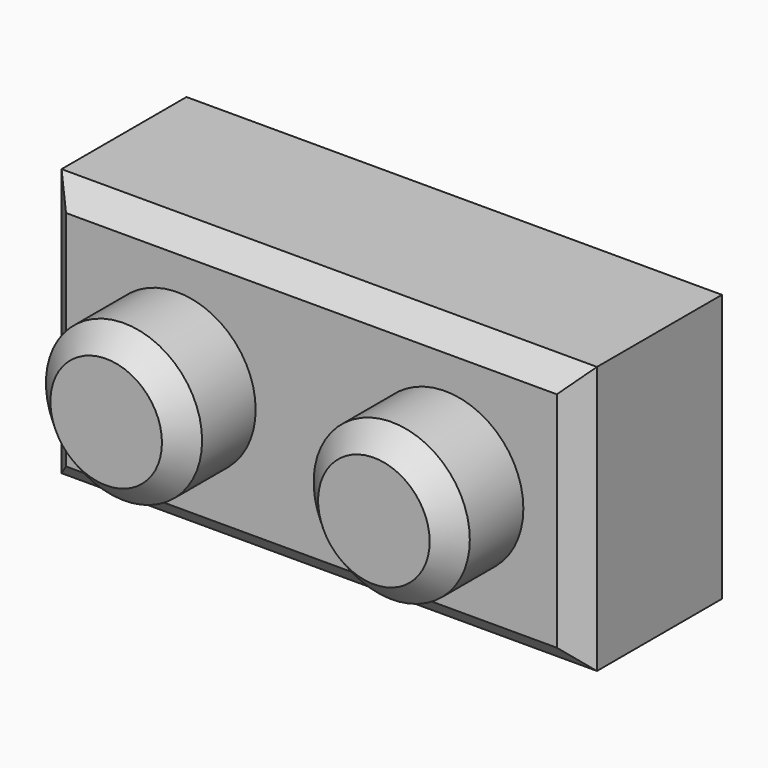
from build123d import *

# Parameters (mm, degrees)
F0_W     = 76.2
F0_H     = 38.1
F1_DEPTH = 25.4
F2_R     = 11.1125
F3_DEPTH = 12.7
F4_SIZE2 = 3.175
F4_SIZE  = 3.175
F5_SIZE2 = 3.175
F5_SIZE  = 3.175
F6_SIZE2 = 3.175
F6_SIZE  = 3.175
F7_T     = 7.9375


# Not quite as in the source:
# - a shell that OpenCascade refuses in one call is made with other operations: the cavity is built on its own and cut out


with BuildPart() as f1:
    # F0 (on Front) → F1 (new body)
    with BuildSketch(Plane.XZ):
        Rectangle(F0_W, F0_H)
    extrude(amount=F1_DEPTH)

    # F2 (on face) → F3 (join)
    with BuildSketch(Plane.XZ.offset(25.4)):
        with Locations((-19.05, 0)):
            Circle(F2_R)
        with Locations((19.05, 0)):
            Circle(F2_R)
    extrude(amount=F3_DEPTH)

    # F4
    f4_edges = [f1.edges().sort_by_distance(p)[0] for p in [
        (7.9375, -38.1, 0),
        (-30.1625, -38.1, 0),
    ]]
    chamfer(f4_edges, length=F4_SIZE, length2=F4_SIZE2)

    # F5
    f5_edges = [f1.edges().sort_by_distance(p)[0] for p in [
        (0, -25.4, 19.05),
    ]]
    chamfer(f5_edges, length=F5_SIZE, length2=F5_SIZE2)

    # F6
    f6_edges = [f1.edges().sort_by_distance(p)[0] for p in [
        (38.1, -25.4, -1.5875),
        (0, -25.4, -19.05),
        (-38.1, -25.4, -1.5875),
    ]]
    chamfer(f6_edges, length=F6_SIZE, length2=F6_SIZE2)

    # F7: shell of thickness 7.9375, made by hand


with BuildPart() as f7_core1:
    # F7_t2: copy of F1
    add(f1.part)

    # the walls: a layer under each face that stays
    f7_faces = [f7_core1.faces().sort_by_distance(p)[0] for p in [
        (0, -25.4, 0),
        (0, -23.8125, 17.4625),
        (36.5125, -23.8125, 0),
        (-36.5125, -23.8125, 0),
        (0, -23.8125, -17.4625),
        (-30.1625, -30.1625, 0),
        (7.9375, -30.1625, 0),
        (0, -11.1125, 19.05),
        (38.1, -11.1125, 0),
        (-38.1, -11.1125, 0),
        (0, -11.1125, -19.05),
        (-28.575, -36.5125, 0),
        (9.525, -36.5125, 0),
        (-19.05, -38.1, 0),
        (19.05, -38.1, 0),
    ]]
    thicken(f7_faces, amount=-F7_T, mode=Mode.SUBTRACT)

    # F7_s3 → F7_t4 (revolve, cut)
    with BuildSketch(Plane.XY):
        Polygon((-7.858125, -25.479375), (-7.9375, -17.4625), (-15.875, -17.4625), (-15.875, -25.4), align=None)
    revolve(axis=Axis((-19.05, -25.4, 0), (0, -1, 0)), mode=Mode.SUBTRACT)

    # F7_s5 → F7_t6 (revolve, cut)
    with BuildSketch(Plane.XY):
        Polygon((30.241875, -25.479375), (30.1625, -17.4625), (22.225, -17.4625), (22.225, -25.4), align=None)
    revolve(axis=Axis((19.05, -25.4, 0), (0, -1, 0)), mode=Mode.SUBTRACT)


with BuildPart() as f1_1:
    add(f1.part)

    # what is left inside the walls is the cavity
    f7_cavity = [f7_core1.part.solids().sort_by_distance(p)[0] for p in [
        (0, -0.079375, -3.704167),
    ]]
    add(f7_cavity, mode=Mode.SUBTRACT)


solid = f1_1.part
